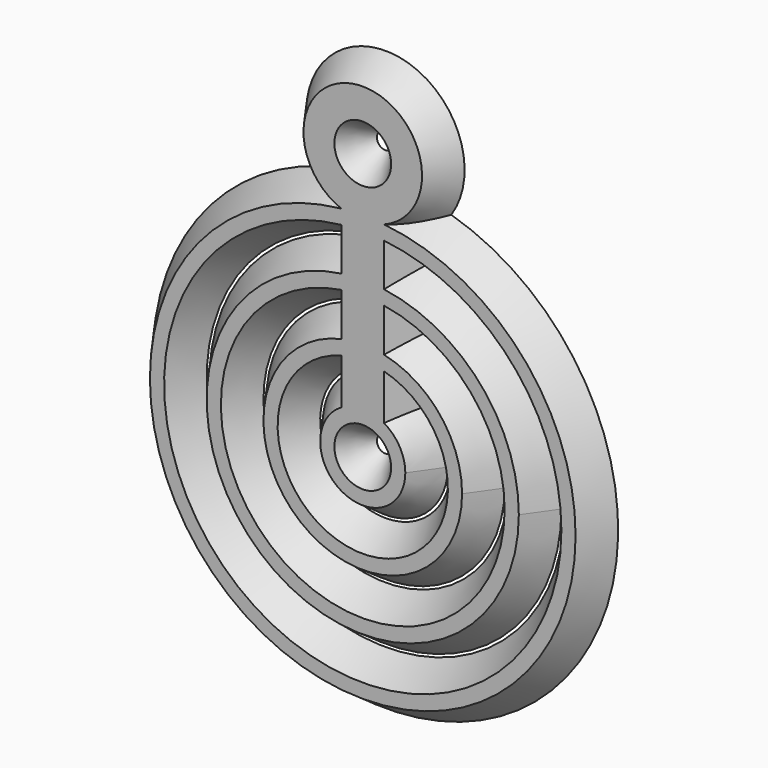
from build123d import *

# Parameters (mm, degrees)
F0_R                   = 6.35
F1_DEPTH               = 6.35
DRAFT_F1_DRAFTED_ANGLE = -35


# Not quite as in the source:
# - an extrude with a draft is written as a straight extrude whose walls are then drafted


with BuildPart() as f1:
    # F0 (on Front) → F1 (new body)
    with BuildSketch(Plane.XZ):
        with BuildLine():
            ThreePointArc((-4.7625000376, 47.3862766884), (-31.9478212145, -35.3196453075), (47.625, 0))
            ThreePointArc((47.625, 0), (35.3196452864, 31.9478212378), (4.7624999752, 47.3862766947))
            ThreePointArc((4.7624999752, 47.3862766947), (-3.14e-08, 47.625), (-4.7625000376, 47.3862766884))
        make_face()
        with BuildLine():
            ThreePointArc((-4.7625000376, 44.1941296259), (-0.0029956665, 44.4499998991), (4.7565431496, 44.194771153))
            ThreePointArc((4.7565431496, 44.194771153), (33.0698566901, 29.7016342732), (44.45, 0))
            ThreePointArc((44.45, 0), (-29.6994054934, -33.071858329), (-4.7625000376, 44.1941296259))
        make_face(mode=Mode.SUBTRACT)
        with BuildLine():
            ThreePointArc((-4.7625000376, 34.5987603592), (-22.9502212537, -26.3257092859), (34.925, 0))
            ThreePointArc((34.925, 0), (26.3237335355, 22.9524873979), (4.7565431496, 34.599579799))
            ThreePointArc((4.7565431496, 34.599579799), (-0.0030064928, 34.9249998706), (-4.7625000376, 34.5987603592))
        make_face()
        with BuildLine():
            ThreePointArc((-4.7625000376, 31.3907803884), (-0.0030124844, 31.7499998571), (4.7565431496, 31.3916835685))
            ThreePointArc((4.7565431496, 31.3916835685), (24.0736655394, 20.7007518583), (31.75, 0))
            ThreePointArc((31.75, 0), (-20.6984676221, -24.0756295473), (-4.7625000376, 31.3907803884))
        make_face(mode=Mode.SUBTRACT)
        with BuildLine():
            ThreePointArc((-4.7625000376, 21.7087359925), (-13.93025595, -17.3175804941), (22.225, 0))
            ThreePointArc((22.225, 0), (17.315669154, 13.9326317237), (4.7565431496, 21.7100419683))
            ThreePointArc((4.7565431496, 21.7100419683), (-0.0030491838, 22.2249997908), (-4.7625000376, 21.7087359925))
        make_face()
        with BuildLine():
            ThreePointArc((-4.7625000376, 18.4450831766), (-0.0030759955, 19.0499997517), (4.7565431496, 18.4466202125))
            ThreePointArc((4.7565431496, 18.4466202125), (15.0584635172, 11.6681265206), (19.05, 0))
            ThreePointArc((19.05, 0), (-11.6656948846, -15.0603473685), (-4.7625000376, 18.4450831766))
        make_face(mode=Mode.SUBTRACT)
        with BuildLine():
            ThreePointArc((-4.7625000376, 47.3862766884), (-3.14e-08, 47.625), (4.7624999752, 47.3862766947))
            ThreePointArc((4.7624999721, 47.3862766632), (3.51e-08, 73.025), (-4.7625000376, 47.3862766884))
        make_face()
        with Locations((0, 59.7633111984)):
            Circle(F0_R, mode=Mode.SUBTRACT)
        with BuildLine():
            ThreePointArc((-4.7625000376, 8.2488919493), (-4.7624999812, -8.2488919819), (9.525, 0))
            ThreePointArc((9.525, 0), (8.2471721972, 4.7654774944), (4.7565431496, 8.2523282936))
            ThreePointArc((4.7565431496, 8.2523282936), (-0.0034384945, 9.5249993794), (-4.7625000376, 8.2488919493))
        make_face()
        Circle(F0_R, mode=Mode.SUBTRACT)
        with BuildLine():
            ThreePointArc((-4.7625000376, 8.2488919493), (-0.0034384945, 9.5249993794), (4.7565431496, 8.2523282936))
            Line((4.7565431496, 8.2523282936), (4.7565431496, 18.4466202125))
            ThreePointArc((4.7565431496, 18.4466202125), (-0.0030759955, 19.0499997517), (-4.7625000376, 18.4450831766))
            Line((-4.7625000376, 18.4450831766), (-4.7625000376, 8.2488919493))
        make_face()
        with BuildLine():
            ThreePointArc((-4.7625000376, 21.7087359925), (-0.0030491838, 22.2249997908), (4.7565431496, 21.7100419683))
            Line((4.7565431496, 21.7100419683), (4.7565431496, 31.3916835685))
            ThreePointArc((4.7565431496, 31.3916835685), (-0.0030124844, 31.7499998571), (-4.7625000376, 31.3907803884))
            Line((-4.7625000376, 31.3907803884), (-4.7625000376, 21.7087359925))
        make_face()
        with BuildLine():
            ThreePointArc((-4.7625000376, 34.5987603592), (-0.0030064928, 34.9249998706), (4.7565431496, 34.599579799))
            Line((4.7565431496, 34.599579799), (4.7565431496, 44.194771153))
            ThreePointArc((4.7565431496, 44.194771153), (-0.0029956665, 44.4499998991), (-4.7625000376, 44.1941296259))
            Line((-4.7625000376, 44.1941296259), (-4.7625000376, 34.5987603592))
        make_face()
    extrude(amount=-F1_DEPTH)

    # draft_F1_drafted
    draft_f1_drafted_walls = [f1.faces().sort_by_distance(p)[0] for p in [
        (3.51e-08, 4.2333333333, 73.025),
        (3.14e-08, 4.2333333333, -47.625),
        (-6.35, 4.2333333333, 59.7633111984),
        (0.0029956665, 4.2333333333, -44.4499998991),
        (-4.7625000376, 4.2333333333, 39.3964449925),
        (0.0030064928, 4.2333333333, -34.9249998706),
        (4.7565431496, 4.2333333333, 39.397175476),
        (-4.7625000376, 4.2333333333, 26.5497581904),
        (0.0030491838, 4.2333333333, -22.2249997908),
        (4.7565431496, 4.2333333333, 26.5508627684),
        (0.0030124844, 4.2333333333, -31.7499998571),
        (0.0030759955, 4.2333333333, -19.0499997517),
        (-4.7625000376, 4.2333333333, 13.346987563),
        (0.0034384945, 4.2333333333, -9.5249993794),
        (4.7565431496, 4.2333333333, 13.3494742531),
        (-6.35, 4.2333333333, 0),
    ]]
    draft(draft_f1_drafted_walls, neutral_plane=Plane(origin=(0, 0, 0), x_dir=(1, 0, 0), z_dir=(0, 1, 0)), angle=DRAFT_F1_DRAFTED_ANGLE)


solid = f1.part
